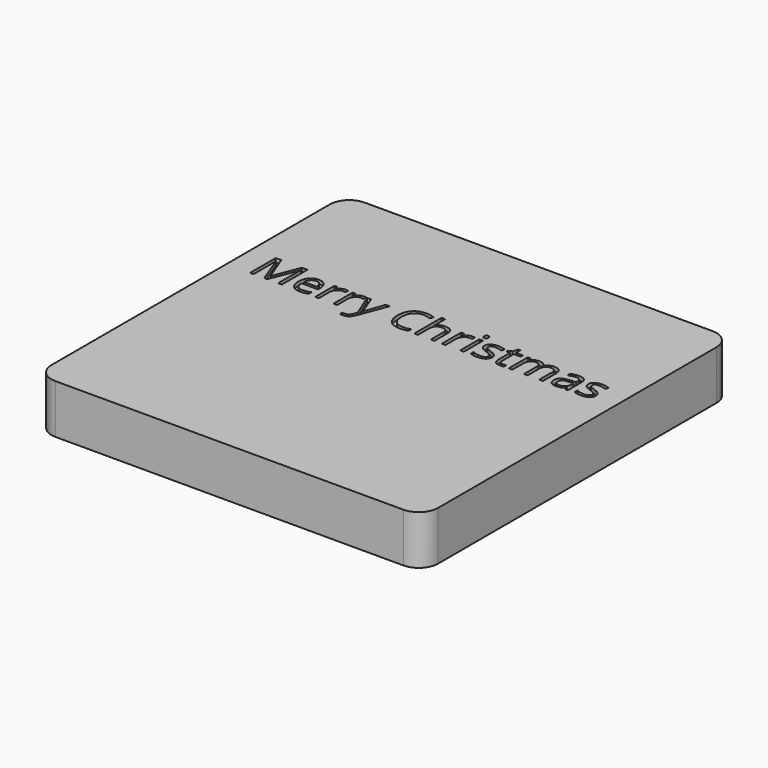
from build123d import *

# Parameters (mm, degrees)
F0_W         = 100
F0_H         = 100
F1_DEPTH     = 12.7
F2_R         = 5
F3_TEXT_SIZE = 11.5944362809
F4_DEPTH     = 1


# Not quite as in the source:
# - Text() gives the source's letters only with a copy of the font that has no kerning and outlines rounded to 1/6400 em; it was checked with that copy


with BuildPart() as f1:
    # F0 (on Top) → F1 (new body)
    with BuildSketch(Plane.XY):
        Rectangle(F0_W, F0_H)
    extrude(amount=F1_DEPTH)

    # F2
    f2_edges = [f1.edges().sort_by_distance(p)[0] for p in [
        (50, -50, 6.35),
        (-50, -50, 6.35),
        (-50, 50, 6.35),
        (50, 50, 6.35),
    ]]
    fillet(f2_edges, radius=F2_R)

    # F3 (on face) → F4 (cut)
    with BuildSketch(Plane.XY.offset(12.7)):
        with Locations((-45, 11.5491598508)):
            Text('Merry Christmas', F3_TEXT_SIZE, font='Open Sans', text_align=(TextAlign.LEFT, TextAlign.BOTTOM))
    extrude(amount=-F4_DEPTH, mode=Mode.SUBTRACT)


solid = f1.part
